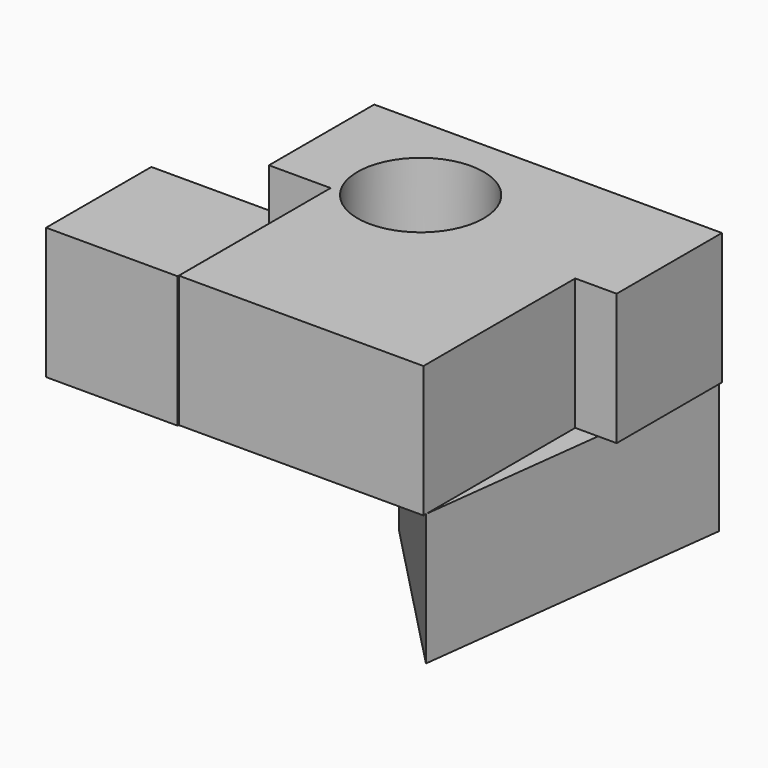
from build123d import *

# Parameters (mm, degrees)
F0_W     = 25.4
F0_H     = 25.4
F1_DEPTH = 25.4
F2_W     = 47.2239479423
F2_H     = 36.629473637
F3_DEPTH = 25.4
F5_DEPTH = 25.4
F6_R     = 12.1699018859
F7_DEPTH = 152.4


# Not quite as in the source:
# - a feature names something its author has since deleted; it is built from what else it names


with BuildPart() as f1:
    # F0 (on Top) → F1 (new body)
    with BuildSketch(Plane.XY):
        with Locations((-58.0832177849, 40.1553949341)):
            Rectangle(F0_W, F0_H)
    extrude(amount=F1_DEPTH)


with BuildPart() as f3:
    # F2 (on face) → F3 (new body)
    with BuildSketch(Plane.XY.offset(25.4)):
        Polygon((40.3320500055, 51.6522369951), (-26.7965224931, 51.6522369951), (-26.7965224931, 26.2522369951), (-14.8890800774, 26.2522369951), (32.3348678648, 26.2522369951), (40.3320500055, 26.2522369951), align=None)
        with Locations((8.7228938937, 7.9375001766)):
            Rectangle(F2_W, F2_H)
    extrude(amount=F3_DEPTH)

    # F4 (on Top) → F5 (join)
    with BuildSketch(Plane.XY):
        Polygon((39.8546084762, 51.5853948891), (-26.9206576049, 51.5853948891), (32.3348678648, -9.7756581381), align=None)
    extrude(amount=F5_DEPTH)

    # F6 (on face) → F7 (cut)
    with BuildSketch(Plane.XY.offset(50.8)):
        with Locations((-2.8575004544, 32.936450094)):
            Circle(F6_R)
    extrude(amount=-F7_DEPTH, mode=Mode.SUBTRACT)


solid = Compound([f1.part, f3.part])
